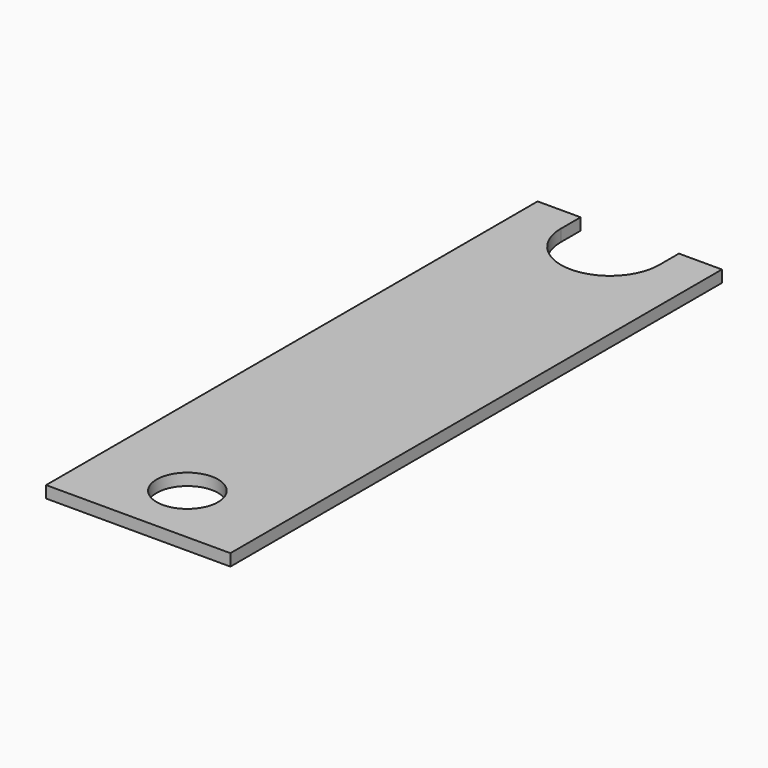
from build123d import *

# Parameters (mm, degrees)
F0_W     = 30
F0_H     = 100
F1_DEPTH = 1.93
F3_D     = 10
F4_DEPTH = 1.93


# Not quite as in the source:
# - a feature names something its author has since deleted; it is built from what else it names


with BuildPart() as f1:
    # F0 (on Top) → F1 (new body)
    with BuildSketch(Plane.XY):
        with Locations((8.4595183283, 3.6650180817)):
            Rectangle(F0_W, F0_H)
    extrude(amount=F1_DEPTH)

    # F3 (through all)
    with Locations(Plane.XY.offset(1.93)):
        with Locations((8.4595183283, -36.3349819183)):
            Hole(F3_D / 2)

    # F2 (on face) → F4 (cut)
    with BuildSketch(Plane.XY.offset(1.93)):
        with BuildLine():
            Line((0.4595183283, 53.6650180817), (0.4595183283, 49.6650180817))
            ThreePointArc((0.4595183283, 49.6650180817), (8.4595183283, 41.6650180817), (16.4595183283, 49.6650180817))
            Line((16.4595183283, 49.6650180817), (16.4595183283, 53.6650180817))
            Line((16.4595183283, 53.6650180817), (0.4595183283, 53.6650180817))
        make_face()
    extrude(amount=-F4_DEPTH, mode=Mode.SUBTRACT)


solid = f1.part
